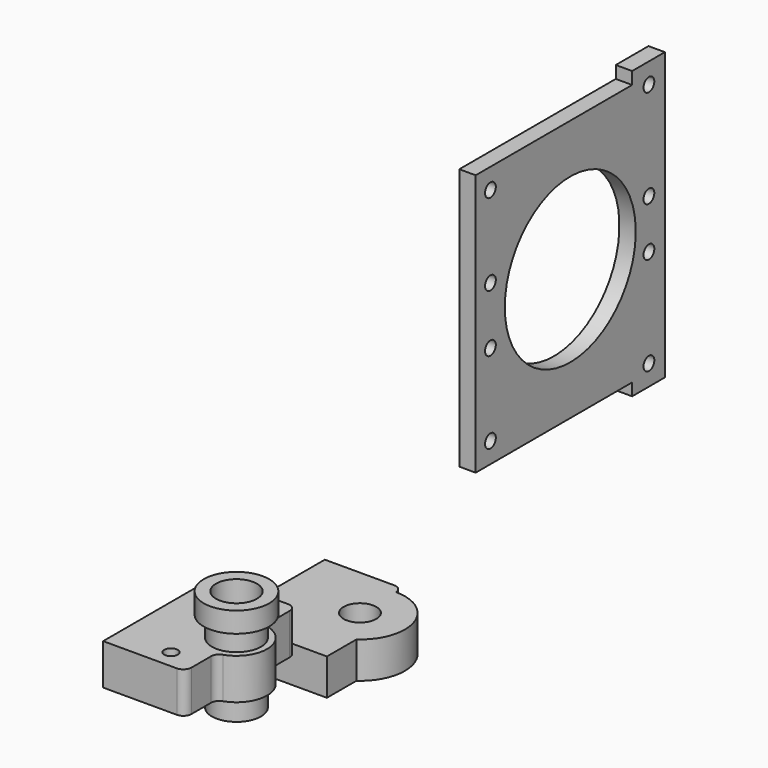
from build123d import *

# Parameters (mm, degrees)
F3_DEPTH  = 10
F4_R      = 2
F5_R      = 2
F6_R      = 6
F7_DEPTH  = 5
F8_R      = 8
F9_DEPTH  = 5
F10_R     = 6
F11_DEPTH = 5
F12_R     = 5
F13_DEPTH = 10
F14_R     = 4
F15_DEPTH = 25
F16_D     = 3.3
F18_D     = 3.3
F18_DEPTH = 5
F18_TIP   = 0.9914200214
F20_DEPTH = 8.9
F21_R     = 1.99999
F22_D     = 8
F24_D     = 3.3
F24_DEPTH = 5
F24_TIP   = 0.9914200214
F25_DEPTH = 64
F26_R     = 20
F27_DEPTH = 33.9511494169
F28_W     = 4
F28_H     = 10
F29_DEPTH = 3
F30_W     = 4
F30_H     = 10
F31_DEPTH = 3
F33_D     = 3.3
F33_DEPTH = 5
F33_TIP   = 0.9914200214


# Not quite as in the source:
# - a fillet or chamfer is up to 0.001 mm smaller than in the source, because OpenCascade refuses the exact size


with BuildPart() as f3:
    # F2 (on Top) → F3 (new body)
    with BuildSketch(Plane.XY):
        with BuildLine():
            Line((167.6959056258, -150.1205759048), (167.6959056258, -184.1205759048))
            Line((167.6959056258, -184.1205759048), (187.6959056258, -184.1205759048))
            Line((187.6959056258, -184.1205759048), (187.6959056258, -174.5519416873))
            ThreePointArc((187.6959056258, -174.5519416873), (194.1835802794, -167.1205759048), (187.6959056258, -159.6892101224))
            Line((187.6959056258, -159.6892101224), (187.6959056258, -150.1205759048))
            Line((187.6959056258, -150.1205759048), (167.6959056258, -150.1205759048))
        make_face()
    extrude(amount=F3_DEPTH)

    # F4
    f4_edges = [f3.edges().sort_by_distance(p)[0] for p in [
        (187.695906, -184.120576, 5),
        (187.695906, -150.120576, 5),
    ]]
    fillet(f4_edges, radius=F4_R)

    # F5
    f5_edges = [f3.edges().sort_by_distance(p)[0] for p in [
        (187.695906, -174.551942, 5),
        (187.695906, -159.68921, 5),
    ]]
    fillet(f5_edges, radius=F5_R)

    # F6 (on face) → F7 (join)
    with BuildSketch(Plane.XY.offset(10)):
        with Locations((186.6835802794, -167.1205759048)):
            Circle(F6_R)
    extrude(amount=F7_DEPTH)

    # F8 (on face) → F9 (join)
    with BuildSketch(Plane.XY.offset(15)):
        with Locations((186.6835802794, -167.1205759048)):
            Circle(F8_R)
    extrude(amount=F9_DEPTH)

    # F10 (on face) → F11 (join)
    with BuildSketch(Plane(origin=(0, 0, 0), x_dir=(1, 0, 0), z_dir=(0, 0, -1))):
        with Locations((186.6835802794, 167.1205759048)):
            Circle(F10_R)
    extrude(amount=F11_DEPTH)

    # F12 (on face) → F13 (cut)
    with BuildSketch(Plane.XY.offset(20)):
        with Locations((186.6835802794, -167.1205759048)):
            Circle(F12_R)
    extrude(amount=-F13_DEPTH, mode=Mode.SUBTRACT)

    # F14 (on face) → F15 (cut, through all)
    with BuildSketch(Plane(origin=(0, 0, -5), x_dir=(1, 0, 0), z_dir=(0, 0, -1))):
        with Locations((186.6835802794, 167.1205759048)):
            Circle(F14_R)
    extrude(amount=-F15_DEPTH, mode=Mode.SUBTRACT)

    # F16 (through all)
    with Locations(Plane(origin=(0, 0, 0), x_dir=(1, 0, 0), z_dir=(0, 0, -1))):
        with Locations((180.6835802794, 179.6205759048), (181.6959056258, 155.1205759048)):
            Hole(F16_D / 2)

    # F18
    with Locations(Plane(origin=(167.6959056258, 0, 0), x_dir=(0, -1, 0), z_dir=(-1, 0, 0))):
        with Locations((155.1205759048, 5), (179.6205759048, 5)):
            Hole(F18_D / 2, depth=F18_DEPTH)
            with Locations((0, 0, -(F18_DEPTH + F18_TIP / 2))):  # 118° drill point
                Cone(0, F18_D / 2, F18_TIP, mode=Mode.SUBTRACT)


with BuildPart() as f20:
    # F19 (on Top) → F20 (new body)
    with BuildSketch(Plane.XY):
        with BuildLine():
            Line((186.6835802794, -116.3909549713), (167.6959056258, -116.3909549713))
            Line((167.6959056258, -116.3909549713), (167.6959056258, -147.3909549713))
            Line((167.6959056258, -147.3909549713), (193.0081355997, -147.3909549713))
            Line((193.0081355997, -147.3909549713), (193.0081355997, -138.3909549713))
            ThreePointArc((193.0081355997, -138.3909549713), (197.1716687611, -126.074330181), (186.6835802794, -118.3909549713))
            Line((186.6835802794, -118.3909549713), (186.6835802794, -116.3909549713))
        make_face()
    extrude(amount=-F20_DEPTH)

    # F21 (radius 2 in the source; OpenCascade refuses exactly that, so slightly less here)
    f21_edges = [f20.edges().sort_by_distance(p)[0] for p in [
        (186.68358, -116.390955, -4.45),
    ]]
    fillet(f21_edges, radius=F21_R)

    # F22 (through all)
    with Locations(Plane.XY):
        with Locations((186.6835802794, -129.3909549713)):
            Hole(F22_D / 2)

    # F24
    with Locations(Plane(origin=(167.6959056258, 0, 0), x_dir=(0, -1, 0), z_dir=(-1, 0, 0))):
        with Locations((121.3909549713, -4.45), (142.3909549713, -4.45)):
            Hole(F24_D / 2, depth=F24_DEPTH)
            with Locations((0, 0, -(F24_DEPTH + F24_TIP / 2))):  # 118° drill point
                Cone(0, F24_D / 2, F24_TIP, mode=Mode.SUBTRACT)


with BuildPart() as f25:
    # F1 (on Top) → F25 (new body)
    with BuildSketch(Plane.XY):
        Polygon((167.7334308624, -70.3457891941), (167.7334308624, -61.3457891941), (167.7334308624, -12.5457891941), (163.7334308624, -12.5457891941), (163.7334308624, -70.3457891941), align=None)
    extrude(amount=F25_DEPTH)

    # F26 (on face) → F27 (cut, through all)
    with BuildSketch(Plane(origin=(163.7334308624, 0, 0), x_dir=(0, -1, 0), z_dir=(-1, 0, 0))):
        with Locations((41.4457891941, 32)):
            Circle(F26_R)
    extrude(amount=-F27_DEPTH, mode=Mode.SUBTRACT)

    # F28 (on face) → F29 (join)
    with BuildSketch(Plane.XY.offset(64)):
        with Locations((165.7334308624, -17.5457891941)):
            Rectangle(F28_W, F28_H)
    extrude(amount=F29_DEPTH)

    # F30 (on face) → F31 (join)
    with BuildSketch(Plane(origin=(0, 0, 0), x_dir=(1, 0, 0), z_dir=(0, 0, -1))):
        with Locations((165.7334308624, 17.5457891941)):
            Rectangle(F30_W, F30_H)
    extrude(amount=F31_DEPTH)

    # F33
    with Locations(Plane(origin=(163.7334308624, 0, 0), x_dir=(0, -1, 0), z_dir=(-1, 0, 0))):
        with Locations((17.4166355282, 2), (17.4166355282, 62), (65.8411160111, 59), (65.8411160111, 5), (17.4166355282, 26), (17.4166355282, 38), (65.8411160111, 25), (65.8411160111, 39)):
            Hole(F33_D / 2, depth=F33_DEPTH)
            with Locations((0, 0, -(F33_DEPTH + F33_TIP / 2))):  # 118° drill point
                Cone(0, F33_D / 2, F33_TIP, mode=Mode.SUBTRACT)


solid = Compound([f3.part, f20.part, f25.part])
